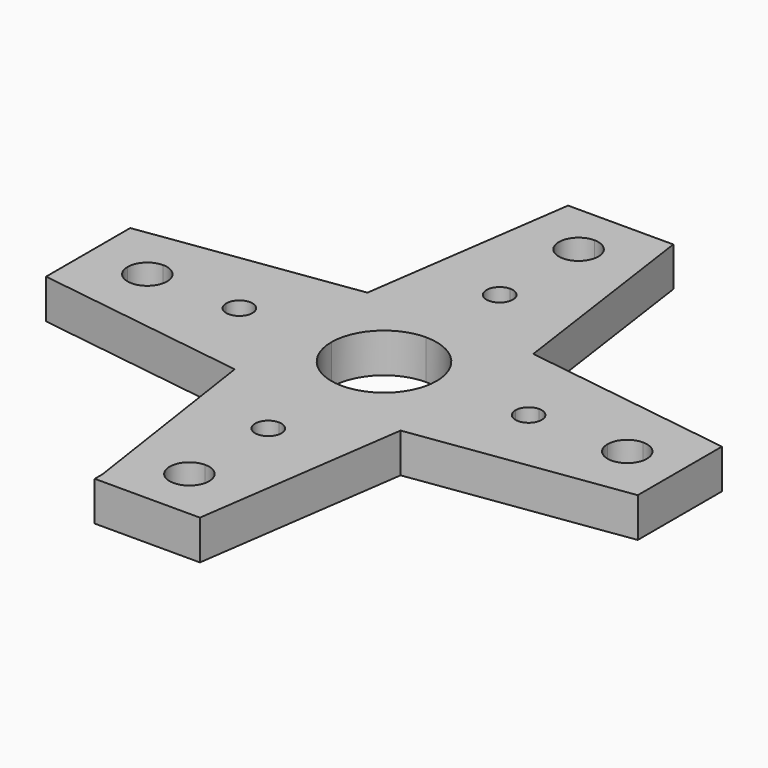
from build123d import *

# Parameters (mm, degrees)
F1_DEPTH = 6


with BuildPart() as f1:
    # F0 (on Top) → F1 (new body)
    with BuildSketch(Plane.XY):
        with BuildLine():
            Line((-4.3394552469, -10.0690543538), (-4.3394552469, -2.0690543538))
            Line((-4.3394552469, -2.0690543538), (-16.3394552469, -2.0690543538))
            ThreePointArc((-16.3394552469, -2.0690543538), (-16.9252416846, -3.4832679161), (-18.3394552469, -4.0690543538))
            ThreePointArc((-18.3394552469, -4.0690543538), (-19.7536688093, -3.4832679161), (-20.3394552469, -2.0690543538))
            Line((-20.3394552469, -2.0690543538), (-29.3394552469, -2.0690543538))
            ThreePointArc((-29.3394552469, -2.0690543538), (-32.3394552469, -5.0690543538), (-35.3394552469, -2.0690543538))
            Line((-35.3394552469, -2.0690543538), (-41.3394552469, -2.0690543538))
            Line((-41.3394552469, -2.0690543538), (-41.3394552469, -5.0690543538))
            Line((-41.3394552469, -5.0690543538), (-41.3394552469, -10.0690543538))
            Line((-41.3394552469, -10.0690543538), (-36.3394552469, -10.0690543538))
            Line((-36.3394552469, -10.0690543538), (-13.5731431865, -10.0690543538))
            Line((-13.5731431865, -10.0690543538), (-13.1868220354, -10.0690543538))
            Line((-13.1868220354, -10.0690543538), (-4.3394552469, -10.0690543538))
        make_face()
        with BuildLine():
            Line((-4.3394552469, 5.9309456462), (-4.3394552469, -2.0690543538))
            ThreePointArc((-4.3394552469, -2.0690543538), (-1.9963094964, 3.5877998957), (3.6605447531, 5.9309456462))
            Line((3.6605447531, 5.9309456462), (-4.3394552469, 5.9309456462))
        make_face()
        with BuildLine():
            ThreePointArc((3.6605447531, -10.0690543538), (-1.9963094964, -7.7259086033), (-4.3394552469, -2.0690543538))
            Line((-4.3394552469, -2.0690543538), (-4.3394552469, -10.0690543538))
            Line((-4.3394552469, -10.0690543538), (3.6605447531, -10.0690543538))
        make_face()
        with BuildLine():
            Line((-16.3394552469, -2.0690543538), (-4.3394552469, -2.0690543538))
            Line((-4.3394552469, -2.0690543538), (-4.3394552469, 5.9309456462))
            Line((-4.3394552469, 5.9309456462), (-11.6972615942, 5.9309456462))
            Line((-11.6972615942, 5.9309456462), (-13.5731431865, 5.9309456462))
            Line((-13.5731431865, 5.9309456462), (-36.3394552469, 5.9309456462))
            Line((-36.3394552469, 5.9309456462), (-41.3394552469, 5.9309456462))
            Line((-41.3394552469, 5.9309456462), (-41.3394552469, 0.9309456462))
            Line((-41.3394552469, 0.9309456462), (-41.3394552469, -2.0690543538))
            Line((-41.3394552469, -2.0690543538), (-35.3394552469, -2.0690543538))
            ThreePointArc((-35.3394552469, -2.0690543538), (-34.4607755905, 0.0522659898), (-32.3394552469, 0.9309456462))
            ThreePointArc((-32.3394552469, 0.9309456462), (-30.2181349034, 0.0522659898), (-29.3394552469, -2.0690543538))
            Line((-29.3394552469, -2.0690543538), (-20.3394552469, -2.0690543538))
            ThreePointArc((-20.3394552469, -2.0690543538), (-18.3394552469, -0.0690543538), (-16.3394552469, -2.0690543538))
        make_face()
        with BuildLine():
            Line((11.6605447531, 5.9309456462), (3.6605447531, 5.9309456462))
            ThreePointArc((3.6605447531, 5.9309456462), (9.3173990026, 3.5877998957), (11.6605447531, -2.0690543538))
            Line((11.6605447531, -2.0690543538), (11.6605447531, 5.9309456462))
        make_face()
        with BuildLine():
            Line((-4.3394552469, 5.9309456462), (3.6605447531, 5.9309456462))
            Line((3.6605447531, 5.9309456462), (3.6605447531, 17.9309456462))
            ThreePointArc((3.6605447531, 17.9309456462), (1.6605447531, 19.9309456462), (3.6605447531, 21.9309456462))
            Line((3.6605447531, 21.9309456462), (3.6605447531, 31.9309456462))
            ThreePointArc((3.6605447531, 31.9309456462), (0.6605447531, 34.9309456462), (3.6605447531, 37.9309456462))
            Line((3.6605447531, 37.9309456462), (3.6605447531, 42.9309456462))
            Line((3.6605447531, 42.9309456462), (0.6605447531, 42.9309456462))
            Line((0.6605447531, 42.9309456462), (-4.3394552469, 42.9309456462))
            Line((-4.3394552469, 42.9309456462), (-4.3394552469, 37.9309456462))
            Line((-4.3394552469, 37.9309456462), (-4.3394552469, 15.1646335859))
            Line((-4.3394552469, 15.1646335859), (-4.3394552469, 14.7783124347))
            Line((-4.3394552469, 14.7783124347), (-4.3394552469, 5.9309456462))
        make_face()
        with BuildLine():
            Line((3.6605447531, 17.9309456462), (3.6605447531, 5.9309456462))
            Line((3.6605447531, 5.9309456462), (11.6605447531, 5.9309456462))
            Line((11.6605447531, 5.9309456462), (11.6605447531, 13.2887519935))
            Line((11.6605447531, 13.2887519935), (11.6605447531, 15.1646335859))
            Line((11.6605447531, 15.1646335859), (11.6605447531, 37.9309456462))
            Line((11.6605447531, 37.9309456462), (11.6605447531, 42.9309456462))
            Line((11.6605447531, 42.9309456462), (6.6605447531, 42.9309456462))
            Line((6.6605447531, 42.9309456462), (3.6605447531, 42.9309456462))
            Line((3.6605447531, 42.9309456462), (3.6605447531, 37.9309456462))
            ThreePointArc((3.6605447531, 37.9309456462), (5.7818650966, 37.0522659898), (6.6605447531, 34.9309456462))
            ThreePointArc((6.6605447531, 34.9309456462), (5.7818650966, 32.8096253027), (3.6605447531, 31.9309456462))
            Line((3.6605447531, 31.9309456462), (3.6605447531, 21.9309456462))
            ThreePointArc((3.6605447531, 21.9309456462), (5.0747583154, 21.3451592086), (5.6605447531, 19.9309456462))
            ThreePointArc((5.6605447531, 19.9309456462), (5.0747583154, 18.5167320839), (3.6605447531, 17.9309456462))
        make_face()
        with BuildLine():
            Line((11.6605447531, -10.0690543538), (3.6605447531, -10.0690543538))
            Line((3.6605447531, -10.0690543538), (3.6605447531, -22.0690543538))
            ThreePointArc((3.6605447531, -22.0690543538), (5.0747583154, -22.6548407914), (5.6605447531, -24.0690543538))
            ThreePointArc((5.6605447531, -24.0690543538), (5.0747583154, -25.4832679161), (3.6605447531, -26.0690543538))
            Line((3.6605447531, -26.0690543538), (3.6605447531, -36.0690543538))
            ThreePointArc((3.6605447531, -36.0690543538), (5.7818650966, -36.9477340102), (6.6605447531, -39.0690543538))
            ThreePointArc((6.6605447531, -39.0690543538), (5.7818650966, -41.1903746973), (3.6605447531, -42.0690543538))
            Line((3.6605447531, -42.0690543538), (3.6605447531, -47.0690543538))
            Line((3.6605447531, -47.0690543538), (6.6605447531, -47.0690543538))
            Line((6.6605447531, -47.0690543538), (11.6605447531, -47.0690543538))
            Line((11.6605447531, -47.0690543538), (11.6605447531, -42.0690543538))
            Line((11.6605447531, -42.0690543538), (11.6605447531, -19.3027422934))
            Line((11.6605447531, -19.3027422934), (11.6605447531, -18.9164211423))
            Line((11.6605447531, -18.9164211423), (11.6605447531, -10.0690543538))
        make_face()
        with BuildLine():
            Line((3.6605447531, -22.0690543538), (3.6605447531, -10.0690543538))
            Line((3.6605447531, -10.0690543538), (-4.3394552469, -10.0690543538))
            Line((-4.3394552469, -10.0690543538), (-4.3394552469, -17.4268607011))
            Line((-4.3394552469, -17.4268607011), (-4.3394552469, -19.3027422934))
            Line((-4.3394552469, -19.3027422934), (-4.3394552469, -42.0690543538))
            Line((-4.3394552469, -42.0690543538), (-4.3394552469, -45.6229187548))
            Line((-4.3394552469, -45.6229187548), (-4.3394552469, -47.0690543538))
            Line((-4.3394552469, -47.0690543538), (0.6605447531, -47.0690543538))
            Line((0.6605447531, -47.0690543538), (3.6605447531, -47.0690543538))
            Line((3.6605447531, -47.0690543538), (3.6605447531, -42.0690543538))
            ThreePointArc((3.6605447531, -42.0690543538), (0.6605447531, -39.0690543538), (3.6605447531, -36.0690543538))
            Line((3.6605447531, -36.0690543538), (3.6605447531, -26.0690543538))
            ThreePointArc((3.6605447531, -26.0690543538), (1.6605447531, -24.0690543538), (3.6605447531, -22.0690543538))
        make_face()
        with BuildLine():
            ThreePointArc((11.6605447531, -2.0690543538), (9.3173990026, -7.7259086033), (3.6605447531, -10.0690543538))
            Line((3.6605447531, -10.0690543538), (11.6605447531, -10.0690543538))
            Line((11.6605447531, -10.0690543538), (11.6605447531, -2.0690543538))
        make_face()
        with BuildLine():
            Line((11.6605447531, 5.9309456462), (11.6605447531, -2.0690543538))
            Line((11.6605447531, -2.0690543538), (23.6605447531, -2.0690543538))
            ThreePointArc((23.6605447531, -2.0690543538), (24.2463311907, -0.6548407914), (25.6605447531, -0.0690543538))
            ThreePointArc((25.6605447531, -0.0690543538), (27.0747583154, -0.6548407914), (27.6605447531, -2.0690543538))
            Line((27.6605447531, -2.0690543538), (37.6605447531, -2.0690543538))
            ThreePointArc((37.6605447531, -2.0690543538), (38.5392244095, 0.0522659898), (40.6605447531, 0.9309456462))
            ThreePointArc((40.6605447531, 0.9309456462), (42.7818650966, 0.0522659898), (43.6605447531, -2.0690543538))
            Line((43.6605447531, -2.0690543538), (48.6605447531, -2.0690543538))
            Line((48.6605447531, -2.0690543538), (48.6605447531, 0.9309456462))
            Line((48.6605447531, 0.9309456462), (48.6605447531, 5.9309456462))
            Line((48.6605447531, 5.9309456462), (43.6605447531, 5.9309456462))
            Line((43.6605447531, 5.9309456462), (20.8942326927, 5.9309456462))
            Line((20.8942326927, 5.9309456462), (20.5079115416, 5.9309456462))
            Line((20.5079115416, 5.9309456462), (11.6605447531, 5.9309456462))
        make_face()
        with BuildLine():
            Line((23.6605447531, -2.0690543538), (11.6605447531, -2.0690543538))
            Line((11.6605447531, -2.0690543538), (11.6605447531, -10.0690543538))
            Line((11.6605447531, -10.0690543538), (19.0183511004, -10.0690543538))
            Line((19.0183511004, -10.0690543538), (20.8942326927, -10.0690543538))
            Line((20.8942326927, -10.0690543538), (43.6605447531, -10.0690543538))
            Line((43.6605447531, -10.0690543538), (48.6605447531, -10.0690543538))
            Line((48.6605447531, -10.0690543538), (48.6605447531, -5.0690543538))
            Line((48.6605447531, -5.0690543538), (48.6605447531, -2.0690543538))
            Line((48.6605447531, -2.0690543538), (43.6605447531, -2.0690543538))
            ThreePointArc((43.6605447531, -2.0690543538), (40.6605447531, -5.0690543538), (37.6605447531, -2.0690543538))
            Line((37.6605447531, -2.0690543538), (27.6605447531, -2.0690543538))
            ThreePointArc((27.6605447531, -2.0690543538), (25.6605447531, -4.0690543538), (23.6605447531, -2.0690543538))
        make_face()
        Polygon((-4.3394552469, -17.4268607011), (-4.3394552469, -10.0690543538), (-13.1868220354, -10.0690543538), (-13.5731431865, -10.0690543538), (-8.9562992167, -14.6858983236), (-4.3394552469, -19.3027422934), align=None)
        Polygon((-11.6972615942, 5.9309456462), (-4.3394552469, 5.9309456462), (-4.3394552469, 14.7783124347), (-4.3394552469, 15.1646335859), (-8.9562992167, 10.547789616), (-13.5731431865, 5.9309456462), align=None)
        Polygon((11.6605447531, 13.2887519935), (11.6605447531, 5.9309456462), (20.5079115416, 5.9309456462), (20.8942326927, 5.9309456462), (16.2773887229, 10.547789616), (11.6605447531, 15.1646335859), align=None)
        Polygon((19.0183511004, -10.0690543538), (11.6605447531, -10.0690543538), (11.6605447531, -18.9164211423), (11.6605447531, -19.3027422934), (16.2773887229, -14.6858983236), (20.8942326927, -10.0690543538), align=None)
        Polygon((-4.3394552469, -42.0690543538), (-4.3394552469, -19.3027422934), (-8.9562992167, -14.6858983236), (-4.3394552469, -45.6229187548), align=None)
        Polygon((-8.9562992167, -14.6858983236), (-13.5731431865, -10.0690543538), (-36.3394552469, -10.0690543538), (-41.3394552469, -10.0690543538), align=None)
        Polygon((-8.9562992167, 10.547789616), (-4.3394552469, 15.1646335859), (-4.3394552469, 37.9309456462), (-4.3394552469, 42.9309456462), align=None)
        Polygon((-36.3394552469, 5.9309456462), (-13.5731431865, 5.9309456462), (-8.9562992167, 10.547789616), (-41.3394552469, 5.9309456462), align=None)
        Polygon((11.6605447531, 37.9309456462), (11.6605447531, 15.1646335859), (16.2773887229, 10.547789616), (11.6605447531, 42.9309456462), align=None)
        Polygon((16.2773887229, 10.547789616), (20.8942326927, 5.9309456462), (43.6605447531, 5.9309456462), (48.6605447531, 5.9309456462), align=None)
        Polygon((16.2773887229, -14.6858983236), (11.6605447531, -19.3027422934), (11.6605447531, -42.0690543538), (11.6605447531, -47.0690543538), align=None)
        Polygon((43.6605447531, -10.0690543538), (20.8942326927, -10.0690543538), (16.2773887229, -14.6858983236), (48.6605447531, -10.0690543538), align=None)
    extrude(amount=-F1_DEPTH)


solid = f1.part
